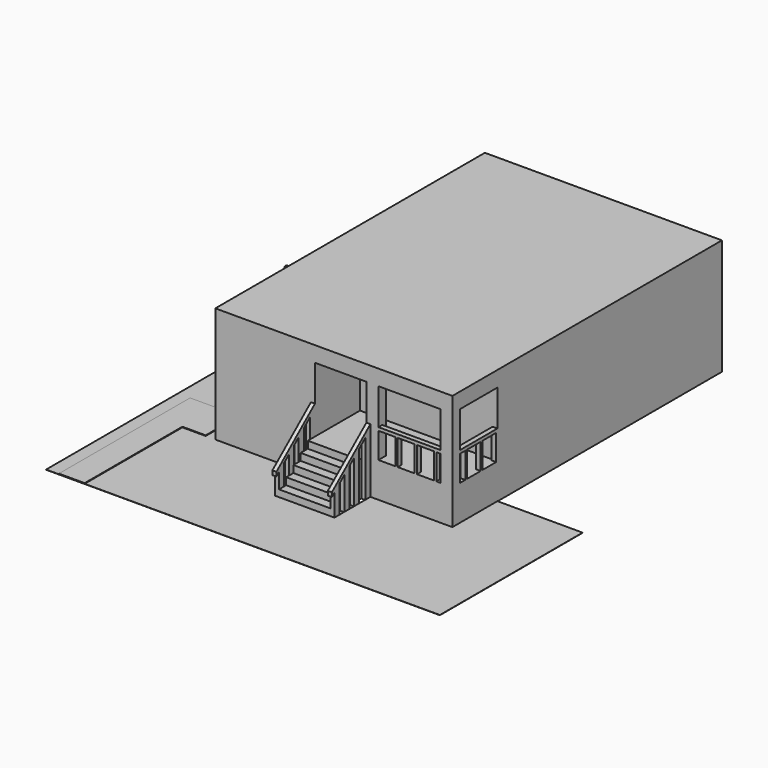
from build123d import *

# Parameters (mm, degrees)
F2_W      = 7493
F2_H      = 10648.549079895
F3_DEPTH  = 3657.6
F4_W      = 4343.4
F4_H      = 2053.1401527691
F5_DEPTH  = 1778
F7_DEPTH  = 914.4
F8_W      = 533.4
F8_H      = 812.8
F9_DEPTH  = 304.8
F10_W     = 533.4
F10_H     = 812.8
F11_DEPTH = 254
F12_W     = 381
F12_H     = 304.8
F13_DEPTH = 2540
F14_W     = 203.2
F14_H     = 812.8
F15_DEPTH = 254
F16_W     = 127
F16_H     = 812.8
F18_DEPTH = 254
F20_DEPTH = 1625.6
F22_DEPTH = 127
F24_W     = 76.2
F24_H     = 1828.8
F25_DEPTH = 2260.6
F26_DEPTH = 25.4
F28_DEPTH = 6.35


# Not quite as in the source:
# - a pattern or mirror of a feature is missing from the dataset's text; its kind, count and spacing are read off the source's solid


with BuildPart() as f3:
    # F2 (on Top) → F3 (new body)
    with BuildSketch(Plane.XY):
        with Locations((3746.5, 5324.2745399475)):
            Rectangle(F2_W, F2_H)
    extrude(amount=F3_DEPTH)

    # F4 (on face) → F5 (cut)
    with BuildSketch(Plane.XZ):
        with Locations((5321.3, 2140.7647186136)):
            Rectangle(F4_W, F4_H)
    extrude(amount=-F5_DEPTH, mode=Mode.SUBTRACT)

    # F6 (on face) → F7 (join)
    with BuildSketch(Plane.XY.offset(1114.1946422291)):
        Polygon((4775.2, 152.4), (4775.2, 0), (7493, 0), (7493, 1778), (7340.6, 1778), (7340.6, 152.4), align=None)
    extrude(amount=F7_DEPTH)

    # F8 (on face) → F9 (cut)
    with BuildSketch(Plane.XZ):
        with Locations((5422.9, 1520.5946422291)):
            Rectangle(F8_W, F8_H)
        with Locations((6032.5, 1520.5946422291)):
            Rectangle(F8_W, F8_H)
        with Locations((6642.1, 1520.5946422291)):
            Rectangle(F8_W, F8_H)
    extrude(amount=-F9_DEPTH, mode=Mode.SUBTRACT)

    # F10 (on face) → F11 (cut)
    with BuildSketch(Plane.YZ.offset(7493)):
        with Locations((1460.5, 1520.5946422291)):
            Rectangle(F10_W, F10_H)
        with Locations((850.9, 1520.5946422291)):
            Rectangle(F10_W, F10_H)
    extrude(amount=-F11_DEPTH, mode=Mode.SUBTRACT)

    # F12 (on face) → F13 (join)
    with BuildSketch(Plane.XY.offset(1114.1946422291)):
        with Locations((4965.7, 152.4)):
            Rectangle(F12_W, F12_H)
        with Locations((7302.5, 152.4)):
            Rectangle(F12_W, F12_H)
    extrude(amount=F13_DEPTH)

    # F14 (on face) → F15 (cut)
    with BuildSketch(Plane.YZ.offset(7493)):
        with Locations((406.4, 1520.5946422291)):
            Rectangle(F14_W, F14_H)
    extrude(amount=-F15_DEPTH, mode=Mode.SUBTRACT)

    # F16 (on face) → F18 (cut)
    with BuildSketch(Plane.XZ):
        with Locations((7048.5, 1520.5946422291)):
            Rectangle(F16_W, F16_H)
    extrude(amount=-F18_DEPTH, mode=Mode.SUBTRACT)

    # F19 (on offset) → F20 (join, through all)
    with BuildSketch(Plane.YZ.offset(3149.6)):
        Polygon((0, 0), (0, 1114.1946422291), (-284.48, 1114.1946422291), (-284.48, 891.3557137833), (-568.96, 891.3557137833), (-568.96, 668.5167853374), (-853.44, 668.5167853374), (-853.44, 445.6778568916), (-1137.92, 445.6778568916), (-1137.92, 222.8389284458), (-1422.4, 222.8389284458), (-1422.4, 0), align=None)
    extrude(amount=F20_DEPTH)

    # F21 (on face) → F22 (join)
    with BuildSketch(Plane(origin=(3149.6, 0, 0), x_dir=(0, -1, 0), z_dir=(-1, 0, 0))):
        Polygon((1524, 751.5465877372), (0, 2030.3344256514), (0, 0), (203.2, 0), (203.2, 1727.2), (441.7354282745, 1527.0450101121), (441.7354282745, 0), (644.9354282745, 0), (644.9354282745, 1356.5399650569), (830.4677141373, 1200.859892418), (830.4677141373, 0), (1033.6677141373, 0), (1033.6677141373, 1030.3548473628), (1219.2, 874.6747747239), (1219.2, 0), (1422.4, 0), (1422.4, 704.1697296687), (1524, 618.917207141), align=None)
    f22 = extrude(amount=F22_DEPTH)

    # F22_copies: F22 across plane
    add(f22.mirror(Plane(origin=(3962.4, 0, 0), x_dir=(0, 0, 1), z_dir=(1, 0, 0))))

    # F24 (on face) → F25 (join, through all)
    with BuildSketch(Plane(origin=(0, 0, 0), x_dir=(0, -1, 0), z_dir=(-1, 0, 0))):
        with Locations((-5600.7, 914.4)):
            Rectangle(F24_W, F24_H)
    extrude(amount=F25_DEPTH)

    # F1 (on Top) → F26 (join)
    with BuildSketch(Plane.XY):
        Polygon((-304.8, 5562.6), (-1498.6, 5562.6), (-1498.6, 4241.8), (-1117.6, 4241.8), (-1117.6, 1320.8), (-1854.2, 1320.8), (-1854.2, -3860.8), (-1041.4, -3860.8), (-1041.4, 0), (-304.8, 0), (-304.8, 4244.8759078979), align=None)
    extrude(amount=F26_DEPTH)

    # F27 (on Top) → F28 (join)
    with BuildSketch(Plane.XY):
        Polygon((0, 5562.6), (-2260.6000000001, 5562.6), (-2260.6000000001, -3860.8), (0, -3860.8), (10185.4, -3860.8), (10185.4, 1778), (7493, 1778), (7493, 0), (4902.2, 0), (4902.2, -1422.4), (4775.2, -1422.4), (3022.6, -1422.4), (3022.6, 0), (0, 0), align=None)
    extrude(amount=F28_DEPTH)


solid = f3.part
